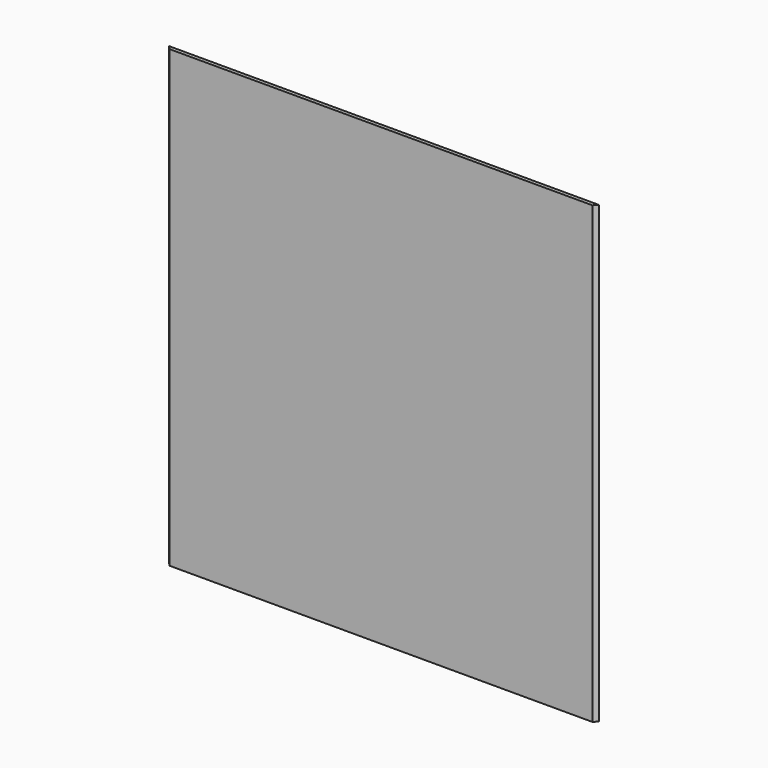
from build123d import *

# Parameters (mm, degrees)
F0_W     = 694
F0_H     = 734
F1_DEPTH = 6
F2_SIZE  = 5.99999


# Not quite as in the source:
# - a fillet or chamfer is up to 0.001 mm smaller than in the source, because OpenCascade refuses the exact size


with BuildPart() as f1:
    # F0 (on Front) → F1 (new body)
    with BuildSketch(Plane.XZ):
        Rectangle(F0_W, F0_H)
    extrude(amount=F1_DEPTH)

    # F2 (size 6 in the source; OpenCascade refuses exactly that, so slightly less here)
    f2_edges = [f1.edges().sort_by_distance(p)[0] for p in [
        (-347, -6, 0),
        (347, -6, 0),
    ]]
    chamfer(f2_edges, length=F2_SIZE)


solid = f1.part
